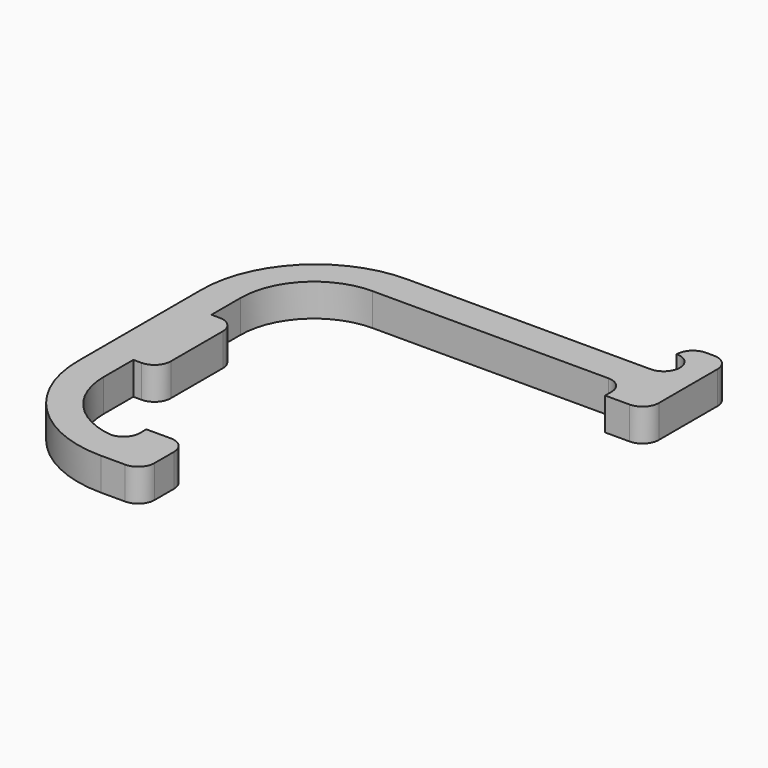
from build123d import *

# Parameters (mm, degrees)
F1_DEPTH    = 4
F2_R        = 1.99999
F3_T1_DEPTH = 4
F4_R        = 14


# Not quite as in the source:
# - a fillet or chamfer that OpenCascade refuses, or shapes differently, is made with other operations: its cross-section is extruded or revolved along the edge and cut away or added
# - a fillet or chamfer is up to 0.001 mm smaller than in the source, because OpenCascade refuses the exact size


with BuildPart() as f1:
    # F0 (on Top) → F1 (new body)
    with BuildSketch(Plane.XY):
        Polygon((32.32, 23.5077), (27.32, 23.5077), (27.32, 20.5077), (17.32, 20.5077), (17.32, 34.0077), (20.32, 34.0077), (20.32, 46.0077), (17.32, 46.0077), (17.32, 59.5077), (57.32, 59.5077), (57.32, 56.5077), (62.32, 56.5077), (62.32, 69.5077), (57.32, 69.5077), (57.32, 67.5077), (59.32, 67.5077), (59.32, 63.5077), (13.32, 63.5077), (13.32, 16.5077), (32.32, 16.5077), align=None)
    extrude(amount=F1_DEPTH)

    # F2 (radius 2 in the source; OpenCascade refuses exactly that, so slightly less here)
    f2_edges = [f1.edges().sort_by_distance(p)[0] for p in [
        (59.32, 63.5077, 2),
        (59.32, 67.5077, 2),
        (57.32, 59.5077, 2),
        (57.32, 69.5077, 2),
        (62.32, 69.5077, 2),
        (62.32, 56.5077, 2),
        (20.32, 46.0077, 2),
        (20.32, 34.0077, 2),
        (27.32, 20.5077, 2),
        (32.32, 16.5077, 2),
        (32.32, 23.5077, 2),
    ]]
    fillet(f2_edges, radius=F2_R)

    # F3: fillet of radius 9 on 2 edges, made by hand

    # F3_s2 → F3_t1 (join)
    with BuildSketch(Plane.XY):
        with BuildLine():
            ThreePointArc((17.32, 50.5077), (19.9560389693, 56.8716610307), (26.32, 59.5077))
            Line((26.32, 59.5077), (26.32, 59.6877))
            Line((26.32, 59.6877), (17.14, 59.6877))
            Line((17.14, 59.6877), (17.14, 50.5077))
            Line((17.14, 50.5077), (17.32, 50.5077))
        make_face()
        with BuildLine():
            ThreePointArc((25.32001, 20.5077), (19.6117994216, 23.451969278), (17.32, 29.451973028))
            Line((17.32, 29.451973028), (17.14, 29.451973028))
            Line((17.14, 29.451973028), (17.14, 20.5077))
            Line((17.14, 20.5077), (17.32, 20.3277))
            ThreePointArc((17.32, 20.3277), (21.320005, 20.3277), (25.3000102, 20.3288145394))
            Line((25.3000102, 20.3288145394), (25.32001, 20.5077))
        make_face()
    extrude(amount=F3_T1_DEPTH)

    # F4
    f4_edges = [f1.edges().sort_by_distance(p)[0] for p in [
        (13.32, 63.5077, 2),
        (13.32, 16.5077, 2),
    ]]
    fillet(f4_edges, radius=F4_R)


solid = f1.part
